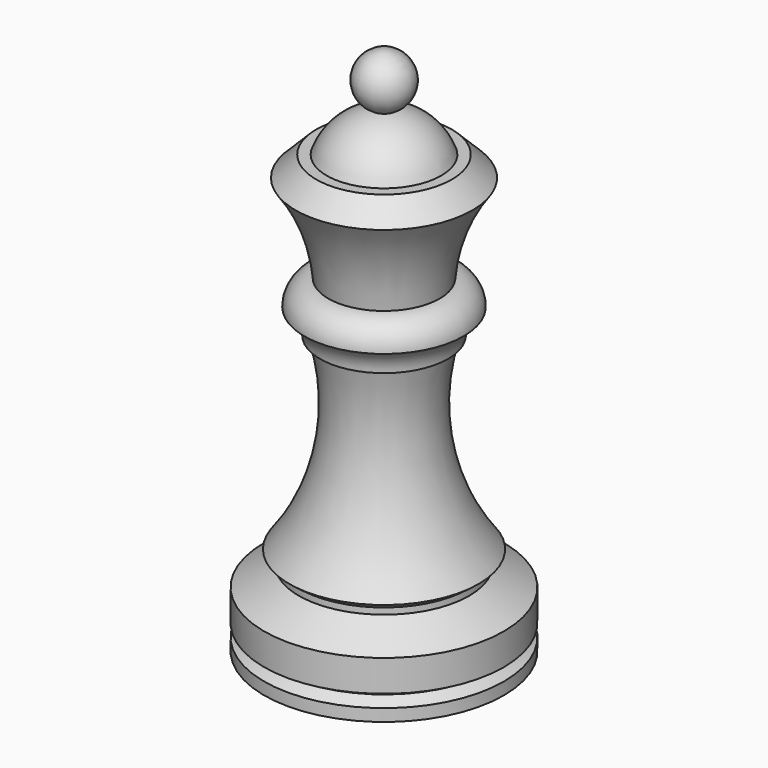
from build123d import *


# Not quite as in the source:
# - a feature names something its author has since deleted; it is built from what else it names


with BuildPart() as f1:
    # F0 (on Front) → F1 (revolve)
    with BuildSketch(Plane.XZ):
        with BuildLine():
            Line((0, 83.9221530378), (0, 52.0721530382))
            Line((0, 52.0721530382), (8.7499442067, 52.0721530382))
            Line((8.7499442067, 52.0721530382), (8.8241037769, 52.0721530382))
            ThreePointArc((8.8241037769, 52.0721530382), (10.4255958993, 59.4368383526), (13.9999442067, 66.0721530382))
            Line((13.9999442067, 66.0721530382), (10.7499442067, 69.3221530382))
            Line((10.7499442067, 69.3221530382), (9.08619756, 69.3221530382))
            ThreePointArc((9.08619756, 69.3221530382), (5.9884215444, 73.6392290372), (1.0750279815, 75.6620797781))
            ThreePointArc((1.0750279815, 75.6620797781), (4.1648192152, 80.2642011572), (0, 83.9221530378))
        make_face()
        with BuildLine():
            Line((0, 52.0721530382), (0, 48.041174956))
            Line((0, 48.041174956), (12.6061004532, 48.041174956))
            ThreePointArc((12.6061004532, 48.041174956), (11.5216028199, 50.8133495764), (8.8241037769, 52.0721530382))
            Line((8.8241037769, 52.0721530382), (8.7499442067, 52.0721530382))
            Line((8.7499442067, 52.0721530382), (0, 52.0721530382))
        make_face()
        with BuildLine():
            Line((0, 48.041174956), (0, 44.0721530382))
            Line((0, 44.0721530382), (9.4, 44.0721530382))
            Line((9.4, 44.0721530382), (10.13, 44.0721530382))
            ThreePointArc((10.13, 44.0721530382), (10.8184777766, 46.3995183881), (12.6061004532, 48.041174956))
            Line((12.6061004532, 48.041174956), (0, 48.041174956))
        make_face()
        Polygon((19, 0), (19, 1.9367265577), (17.2679491924, 2.9367265577), (19, 3.9367265577), (19, 8.9367265577), (13.5, 12.1121530382), (0, 12.1121530382), (0, 0), align=None)
        with BuildLine():
            Line((0, 44.0721530382), (0, 12.1121530382))
            Line((0, 12.1121530382), (13.5, 12.1121530382))
            Line((13.5, 12.1121530382), (13.5, 13.1121530382))
            Line((13.5, 13.1121530382), (15, 14.2461276344))
            ThreePointArc((15, 14.2461276344), (8.6430304158, 28.4912997708), (9.4, 44.0721530382))
            Line((9.4, 44.0721530382), (0, 44.0721530382))
        make_face()
    revolve(axis=Axis((0, 0, 41.9610765189), (0, 0, -1)))


solid = f1.part
